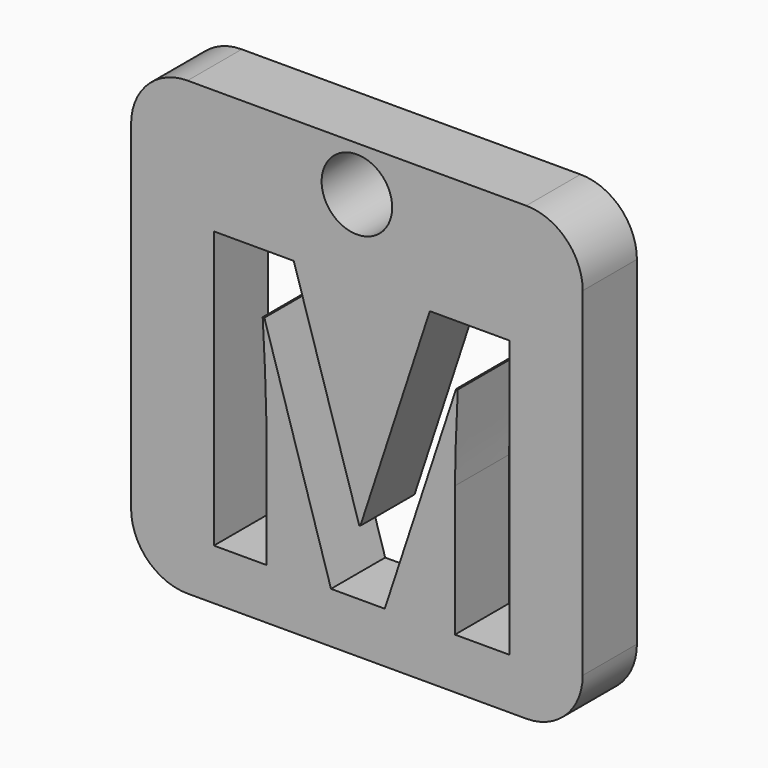
from build123d import *

# Parameters (mm, degrees)
F0_W         = 20.32
F0_H         = 20.32
F1_DEPTH     = 3.048
F2_R         = 2.54
F3_R         = 1.5875
F5_DEPTH     = 25.4
F6_TEXT_SIZE = 17.4349336057
F7_DEPTH     = 25.4


# Not quite as in the source:
# - Text() gives the source's letters only with a copy of the font that has no kerning and outlines rounded to 1/6400 em; it was checked with that copy


with BuildPart() as f1:
    # F0 (on Front) → F1 (new body)
    with BuildSketch(Plane.XZ):
        with Locations((10.16, 10.16)):
            Rectangle(F0_W, F0_H)
    extrude(amount=F1_DEPTH)

    # F2
    f2_edges = [f1.edges().sort_by_distance(p)[0] for p in [
        (20.32, -1.524, 20.32),
        (0, -1.524, 0),
        (0, -1.524, 20.32),
        (20.32, -1.524, 0),
    ]]
    fillet(f2_edges, radius=F2_R)

    # F3 (on Front) → F5 (cut)
    with BuildSketch(Plane.XZ):
        with Locations((10.16, 18.2881587252)):
            Circle(F3_R)
    extrude(amount=F5_DEPTH, mode=Mode.SUBTRACT)

    # F6 (on offset) → F7 (cut)
    with BuildSketch(Plane.XZ.offset(25.4)):
        with Locations((2.159, 2.286)):
            Text('M', F6_TEXT_SIZE, font='Open Sans', font_style=FontStyle.BOLD, text_align=(TextAlign.LEFT, TextAlign.BOTTOM))
    extrude(amount=-F7_DEPTH, mode=Mode.SUBTRACT)


solid = f1.part
